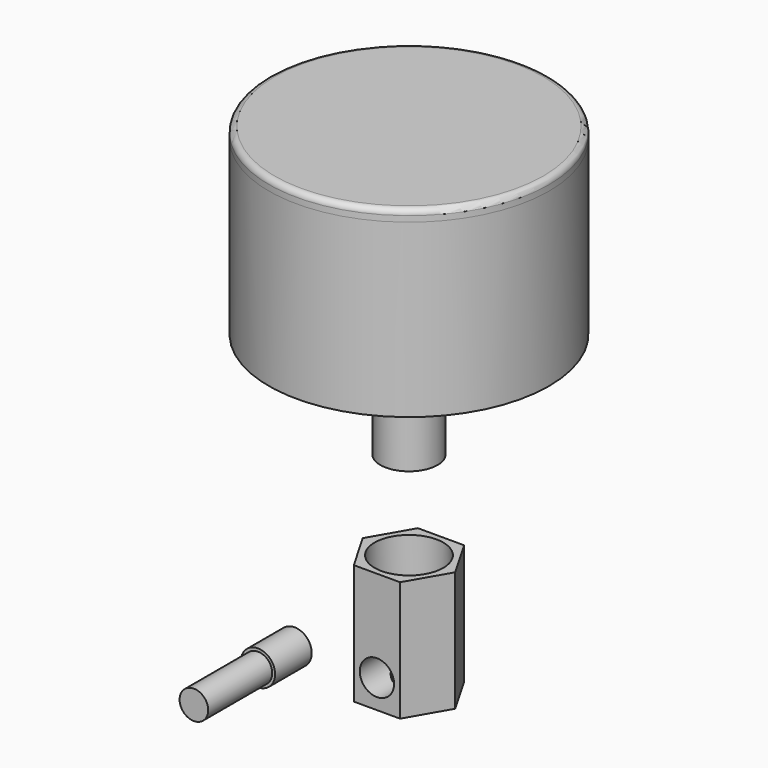
from build123d import *
from build123d import SkipClean  # not in build123d's __all__

# Parameters (mm, degrees)
F0_R      = 24.5
F1_DEPTH  = 30
F2_R      = 5
F3_DEPTH  = 18.5
F6_DEPTH  = 21
F7_R      = 6
F8_DEPTH  = 10
F9_R      = 2.5
F10_DEPTH = 9
F11_R     = 3
F12_DEPTH = 7
F14_R     = 3
F15_DEPTH = 8
F16_R     = 2.5
F17_DEPTH = 14
F18_R     = 24.5
F19_DEPTH = 2
F20_R     = 1


with BuildPart() as f1:
    # F0 (on Top) → F1 (new body)
    with BuildSketch(Plane.XY):
        Circle(F0_R)
    extrude(amount=F1_DEPTH)


with BuildPart() as f3:
    # F2 (on face) → F3 (new body)
    with BuildSketch(Plane(origin=(0, 0, 0), x_dir=(1, 0, 0), z_dir=(0, 0, -1))):
        Circle(F2_R)
    extrude(amount=F3_DEPTH)


with BuildPart() as f6:
    # F5 (on offset) → F6 (new body)
    with BuildSketch(Plane.XY.offset(-55)):
        Polygon((4.0414518843, 7), (-4.0414518843, 7), (-8.0829037687, 0), (-4.0414518843, -7), (4.0414518843, -7), (8.0829037687, 0), align=None)
    extrude(amount=F6_DEPTH)

    # F7 (on face) → F8 (cut)
    with BuildSketch(Plane.XY.offset(-34)):
        Circle(F7_R)
    extrude(amount=-F8_DEPTH, mode=Mode.SUBTRACT)

    # F9 (on face) → F10 (cut)
    with BuildSketch(Plane.XY.offset(-44)):
        Circle(F9_R)
    extrude(amount=-F10_DEPTH, mode=Mode.SUBTRACT)

    # F11 (on face) → F12 (cut)
    with BuildSketch(Plane.XZ.offset(7)):
        with Locations((0, -50)):
            Circle(F11_R)
    with SkipClean():  # cleaning this boolean's faces spoils the solid; the shape is the same uncleaned
        extrude(amount=-F12_DEPTH, mode=Mode.SUBTRACT)


with BuildPart() as f15:
    # F14 (on offset) → F15 (new body)
    with BuildSketch(Plane.XZ.offset(25)):
        with Locations((0, -37.9232009678)):
            Circle(F14_R)
    extrude(amount=F15_DEPTH)

    # F16 (on face) → F17 (join)
    with BuildSketch(Plane.XZ.offset(33)):
        with Locations((0, -37.9232009678)):
            Circle(F16_R)
    extrude(amount=F17_DEPTH)


with BuildPart() as f19:
    # F18 (on face) → F19 (new body)
    with BuildSketch(Plane.XY.offset(30)):
        Circle(F18_R)
    extrude(amount=F19_DEPTH)

    # F20
    f20_edges = [f19.edges().sort_by_distance(p)[0] for p in [
        (-24.5, 0, 32),
    ]]
    fillet(f20_edges, radius=F20_R)


solid = Compound([f1.part, f3.part, f6.part, f15.part, f19.part])
